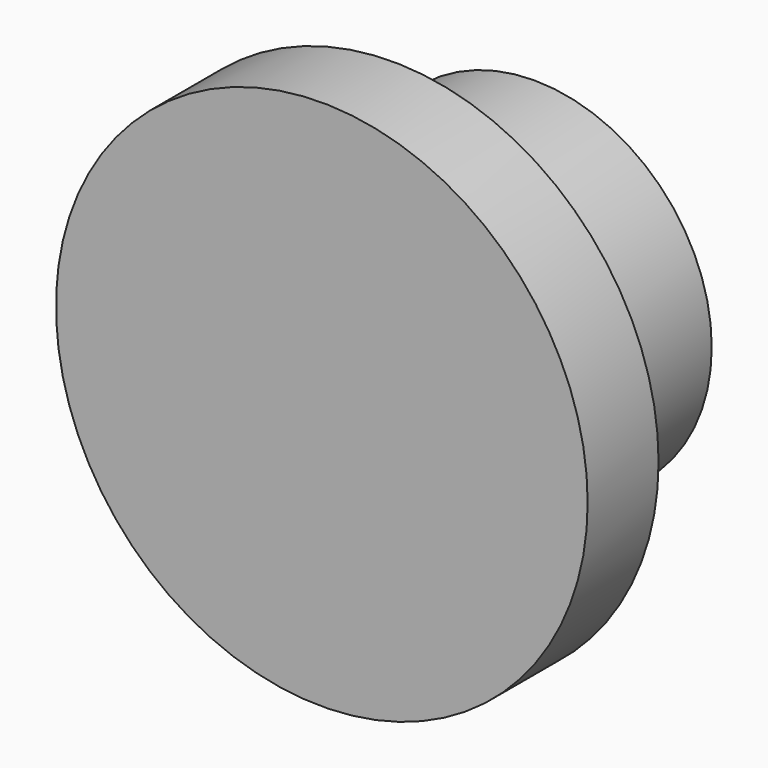
from build123d import *

# Parameters (mm, degrees)
F0_R     = 12.7
F1_DEPTH = 12.7
F2_R     = 19.05
F2_R_2   = 12.7
F3_DEPTH = 6.35


with BuildPart() as f1:
    # F0 (on Front) → F1 (new body)
    with BuildSketch(Plane.XZ):
        Circle(F0_R)
    extrude(amount=F1_DEPTH)

    # F2 (on face) → F3 (join)
    with BuildSketch(Plane.XZ.offset(12.7)):
        Circle(F2_R)
        Circle(F2_R_2, mode=Mode.SUBTRACT)
        Circle(F2_R_2)
    extrude(amount=F3_DEPTH)


solid = f1.part
